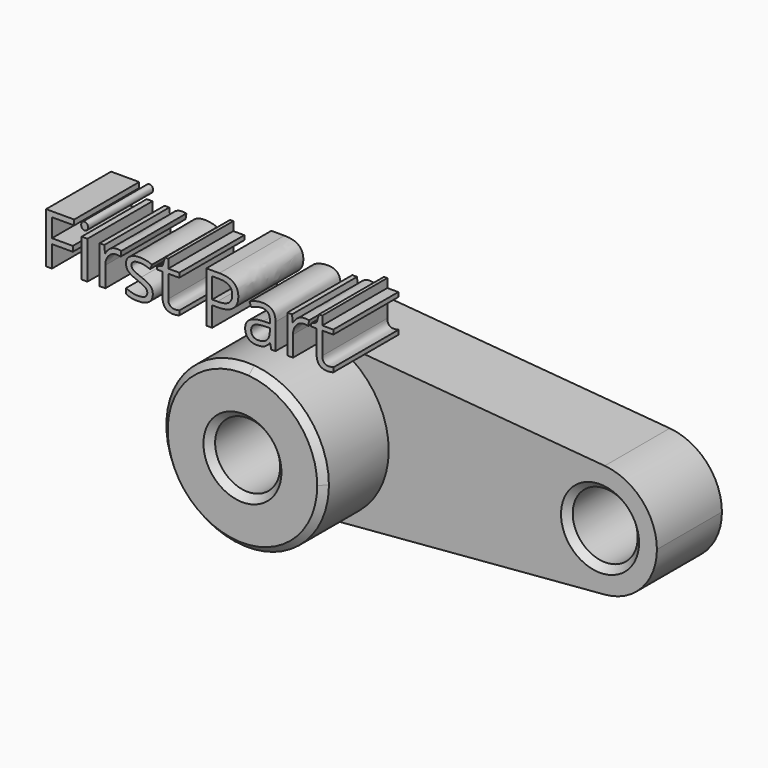
from build123d import *

# Parameters (mm, degrees)
F0_R         = 10
F1_DEPTH     = 25
F2_DEPTH     = 50
F3_SIZE      = 2
F5_START     = 25
F4_TEXT_SIZE = 21.7413115833
F5_DEPTH     = 25


# Not quite as in the source:
# - Text() gives the source's letters only with a copy of the font that has no kerning and outlines rounded to 1/6400 em; it was checked with that copy


with BuildPart() as f1:
    # F0 (on Front) → F1 (new body)
    with BuildSketch(Plane.XZ):
        with BuildLine():
            ThreePointArc((2.0833333333, -24.9130432148), (18.3995018048, -16.9250800097), (25, 0))
            ThreePointArc((25, 0), (18.3995018048, 16.9250800097), (2.0833333333, 24.9130432148))
            ThreePointArc((2.0833333333, 24.9130432148), (-25, 0), (2.0833333333, -24.9130432148))
        make_face()
        Circle(F0_R, mode=Mode.SUBTRACT)
        with BuildLine():
            ThreePointArc((2.0833333333, 24.9130432148), (18.3995018048, 16.9250800097), (25, 0))
            ThreePointArc((25, 0), (18.3995018048, -16.9250800097), (2.0833333333, -24.9130432148))
            Line((2.0833333333, -24.9130432148), (91.4583333333, -17.4391302504))
            ThreePointArc((91.4583333333, -17.4391302504), (72.5, 0), (91.4583333333, 17.4391302504))
            Line((91.4583333333, 17.4391302504), (2.0833333333, 24.9130432148))
        make_face()
        with BuildLine():
            ThreePointArc((107.5, 0), (102.8796512634, 11.8475560068), (91.4583333333, 17.4391302504))
            ThreePointArc((91.4583333333, 17.4391302504), (72.5, 0), (91.4583333333, -17.4391302504))
            ThreePointArc((91.4583333333, -17.4391302504), (102.8796512634, -11.8475560068), (107.5, 0))
        make_face()
        with Locations((90, 0)):
            Circle(F0_R, mode=Mode.SUBTRACT)
    extrude(amount=F1_DEPTH)

    # F0 (on Front) → F2 (join)
    with BuildSketch(Plane.XZ):
        with BuildLine():
            ThreePointArc((2.0833333333, -24.9130432148), (18.3995018048, -16.9250800097), (25, 0))
            ThreePointArc((25, 0), (18.3995018048, 16.9250800097), (2.0833333333, 24.9130432148))
            ThreePointArc((2.0833333333, 24.9130432148), (-25, 0), (2.0833333333, -24.9130432148))
        make_face()
        Circle(F0_R, mode=Mode.SUBTRACT)
    extrude(amount=F2_DEPTH)

    # F3
    f3_edges = [f1.edges().sort_by_distance(p)[0] for p in [
        (-2.083333, -50, 24.913043),
        (-10, -50, 0),
        (80, -25, 0),
    ]]
    chamfer(f3_edges, length=F3_SIZE)


with BuildPart() as f5:
    # F4 (on Front) → F5 (new body)
    with BuildSketch(Plane.XZ.offset(F5_START)):
        with Locations((-62.5382810831, 32.2072990239)):
            Text('First Part', F4_TEXT_SIZE, font='Open Sans', text_align=(TextAlign.LEFT, TextAlign.BOTTOM))
    extrude(amount=F5_DEPTH)


solid = Compound([f1.part, f5.part])
